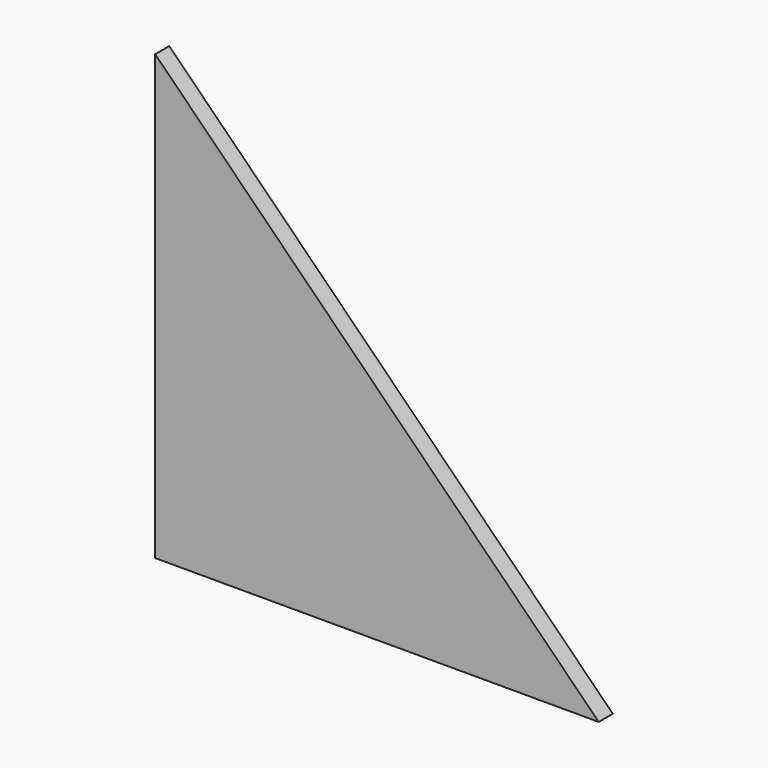
from build123d import *

# Parameters (mm, degrees)
F1_DEPTH = 1.5875


# Not quite as in the source:
# - a length typed as a fraction of an inch, garbled in the dataset ("3 / 203.2 mm" for 3/8 in), is restored


with BuildPart() as f1:
    # F0 (on Front) → F1 (new body, symmetric)
    with BuildSketch(Plane.XZ):
        Polygon((0, 80), (0, 0), (80, 0), align=None)
    extrude(amount=F1_DEPTH, both=True)


solid = f1.part
